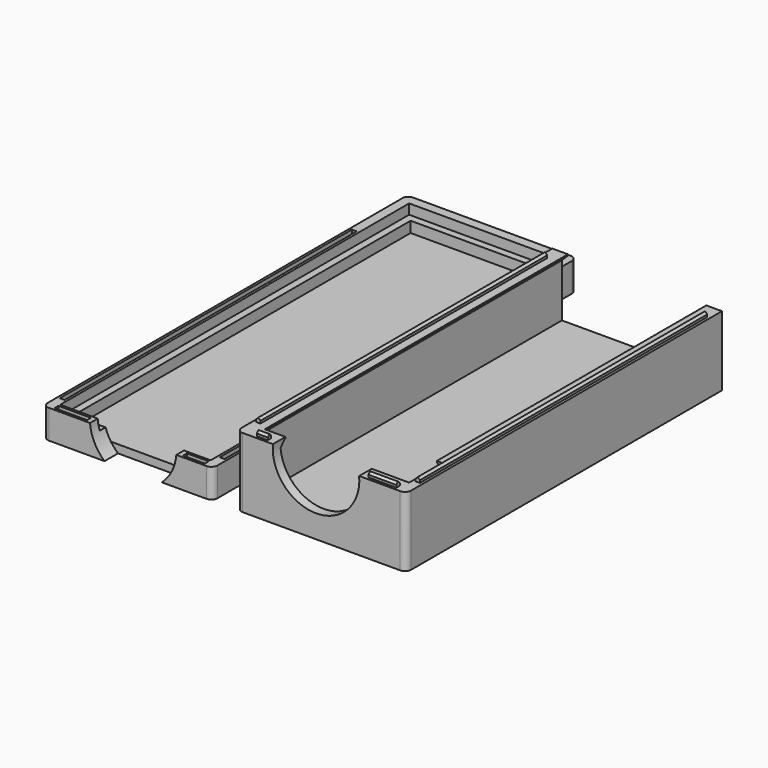
from build123d import *

# Parameters (mm, degrees)
F0_W         = 35.814
F0_H         = 96.139
F1_DEPTH     = 6.096
F2_W         = 28.702
F2_H         = 89.027
F3_DEPTH     = 4.3942
F4_W         = 31.75
F4_H         = 92.075
F4_W_2       = 28.702
F4_H_2       = 89.027
F5_DEPTH     = 2.1082
F6_W         = 35.814
F6_H         = 96.012
F7_DEPTH     = 14.732
F8_T         = -2.032
F9_W         = 35.814
F9_H         = 12.7
F9_W_2       = 10.16
F9_H_2       = 8.89
F9_R         = 3.175
F10_DEPTH    = 14.733
F11_W        = 1.27
F11_H        = 71.12
F12_DEPTH    = 1.524
F13_SIZE     = 1.26999
F14_R        = 1.27
F14_2_R      = 1.27
F15_R        = 9.144
F16_DEPTH    = 96.14
F17_DEPTH    = 3.556
F18_W        = 6.8898053138
F18_H        = 1.016
F18_W_2      = 1.016
F18_H_2      = 77.089
F18_W_3      = 4.6038053138
F19_DEPTH    = 1.016
F20_W        = 2.3178053138
F20_H        = 0.9144
F20_W_2      = 0.9144
F20_H_2      = 75.692
F20_W_3      = 5.8738053138
F20_H_3      = 75.819
F21_DEPTH    = 1.143
F22_T1_DEPTH = 5.5838427085
F22_T3_DEPTH = 78.9580373947
F22_T5_DEPTH = 9.1398427085
F22_T7_DEPTH = 79.0850373947


# Not quite as in the source:
# - a fillet or chamfer that OpenCascade refuses, or shapes differently, is made with other operations: its cross-section is extruded or revolved along the edge and cut away or added
# - a fillet or chamfer is up to 0.001 mm smaller than in the source, because OpenCascade refuses the exact size
# - a feature names something its author has since deleted; it is built from what else it names


with BuildPart() as f1:
    # F0 (on Top) → F1 (new body)
    with BuildSketch(Plane.XY):
        with Locations((20.447, 50.6095)):
            Rectangle(F0_W, F0_H)
    extrude(amount=F1_DEPTH)

    # F2 (on face) → F3 (cut)
    with BuildSketch(Plane.XY.offset(6.096)):
        with Locations((20.447, 50.6095)):
            Rectangle(F2_W, F2_H)
    extrude(amount=-F3_DEPTH, mode=Mode.SUBTRACT)

    # F4 (on face) → F5 (cut)
    with BuildSketch(Plane.XY.offset(6.096)):
        with Locations((20.447, 50.6095)):
            Rectangle(F4_W, F4_H)
        with Locations((20.447, 50.6095)):
            Rectangle(F4_W_2, F4_H_2, mode=Mode.SUBTRACT)
    extrude(amount=-F5_DEPTH, mode=Mode.SUBTRACT)

    # F14
    f14_edges = [f1.edges().sort_by_distance(p)[0] for p in [
        (38.354, 2.54, 3.048),
        (38.354, 98.679, 3.048),
        (2.54, 2.54, 3.048),
        (2.54, 98.679, 3.048),
    ]]
    fillet(f14_edges, radius=F14_R)

    # F15 (on face) → F17 (cut)
    with BuildSketch(Plane.XZ.offset(-2.54)):
        with Locations((60.198, 13.97)):
            Circle(F15_R)
        with Locations((21.59, 6.858)):
            Circle(F15_R)
    extrude(amount=-F17_DEPTH, mode=Mode.SUBTRACT)

    # F18 (on face) → F19 (cut)
    with BuildSketch(Plane.XY.offset(6.096)):
        with Locations((8.0169026569, 3.556)):
            Rectangle(F18_W, F18_H)
        with Locations((3.556, 44.8945)):
            Rectangle(F18_W_2, F18_H_2)
        with Locations((37.338, 44.8945)):
            Rectangle(F18_W_2, F18_H_2)
        with Locations((34.0200973431, 3.556)):
            Rectangle(F18_W_3, F18_H)
    extrude(amount=-F19_DEPTH, mode=Mode.SUBTRACT)


with BuildPart() as f7:
    # F6 (on Top) → F7 (new body)
    with BuildSketch(Plane.XY):
        with Locations((61.341, 50.546)):
            Rectangle(F6_W, F6_H)
    extrude(amount=F7_DEPTH)

    # F8
    f8_openings = [f7.faces().sort_by_distance(p)[0] for p in [
        (61.341, 50.546, 14.732),
    ]]
    offset(amount=F8_T, openings=f8_openings)

    # F9 (on face) → F10 (cut, through all)
    with BuildSketch(Plane.XY.offset(14.732)):
        with Locations((61.341, 92.202)):
            Rectangle(F9_W, F9_H)
        with Locations((72.136, 9.017)):
            Rectangle(F9_W_2, F9_H_2)
        with Locations((64.389, 45.466)):
            Circle(F9_R)
    extrude(amount=-F10_DEPTH, mode=Mode.SUBTRACT)

    # F11 (on face) → F12 (join)
    with BuildSketch(Plane.XY.offset(14.732)):
        with Locations((76.581, 50.292)):
            Rectangle(F11_W, F11_H)
        Polygon((45.466, 85.852), (45.466, 4.572), (77.216, 4.572), (77.216, 5.842), (46.736, 5.842), (46.736, 85.852), align=None)
    extrude(amount=-F12_DEPTH)

    # F13 (size 1.27 in the source; OpenCascade refuses exactly that, so slightly less here)
    f13_edges = [f7.edges().sort_by_distance(p)[0] for p in [
        (61.976, 5.842, 13.208),
        (75.946, 50.292, 13.208),
        (46.736, 45.847, 13.208),
    ]]
    chamfer(f13_edges, length=F13_SIZE)

    # F14#2
    f14_2_edges = [f7.edges().sort_by_distance(p)[0] for p in [
        (79.248, 2.54, 7.366),
        (43.434, 2.54, 7.366),
    ]]
    fillet(f14_2_edges, radius=F14_2_R)

    # F15 (on face) → F16 (cut, through all)
    with BuildSketch(Plane.XZ.offset(-2.54)):
        with Locations((60.198, 13.97)):
            Circle(F15_R)
        with Locations((21.59, 6.858)):
            Circle(F15_R)
    extrude(amount=-F16_DEPTH, mode=Mode.SUBTRACT)

    # F20 (on face) → F21 (join)
    with BuildSketch(Plane.XY.offset(14.732)):
        with Locations((48.4029026569, 3.556)):
            Rectangle(F20_W, F20_H)
        with Locations((44.45, 44.831)):
            Rectangle(F20_W_2, F20_H_2)
        with Locations((73.7710973431, 3.556)):
            Rectangle(F20_W_3, F20_H)
        with Locations((78.232, 44.7675)):
            Rectangle(F20_W_2, F20_H_3)
    extrude(amount=F21_DEPTH)

    # F22: chamfer of 0.635 on 8 edges, made by hand

    # F22_s2 → F22_t1 (cut)
    with BuildSketch(Plane.YZ.offset(45.6109813026)):
        Polygon((3.0988, 15.24), (3.7338, 15.875), (3.0988, 15.875), align=None)
        Polygon((4.0132, 15.24), (3.3782, 15.875), (4.0132, 15.875), align=None)
    extrude(amount=F22_T1_DEPTH, mode=Mode.SUBTRACT)

    # F22_s4 → F22_t3 (cut)
    with BuildSketch(Plane.XZ.offset(-84.3100186974)):
        Polygon((44.9072, 15.24), (44.2722, 15.875), (44.9072, 15.875), align=None)
        Polygon((43.9928, 15.24), (44.6278, 15.875), (43.9928, 15.875), align=None)
    extrude(amount=F22_T3_DEPTH, mode=Mode.SUBTRACT)

    # F22_s6 → F22_t5 (cut)
    with BuildSketch(Plane.YZ.offset(69.2011759889)):
        Polygon((3.0988, 15.24), (3.7338, 15.875), (3.0988, 15.875), align=None)
        Polygon((4.0132, 15.24), (3.3782, 15.875), (4.0132, 15.875), align=None)
    extrude(amount=F22_T5_DEPTH, mode=Mode.SUBTRACT)

    # F22_s8 → F22_t7 (cut)
    with BuildSketch(Plane.XZ.offset(-84.3100186974)):
        Polygon((78.6892, 15.24), (78.0542, 15.875), (78.6892, 15.875), align=None)
        Polygon((77.7748, 15.24), (78.4098, 15.875), (77.7748, 15.875), align=None)
    extrude(amount=F22_T7_DEPTH, mode=Mode.SUBTRACT)


solid = Compound([f1.part, f7.part])
